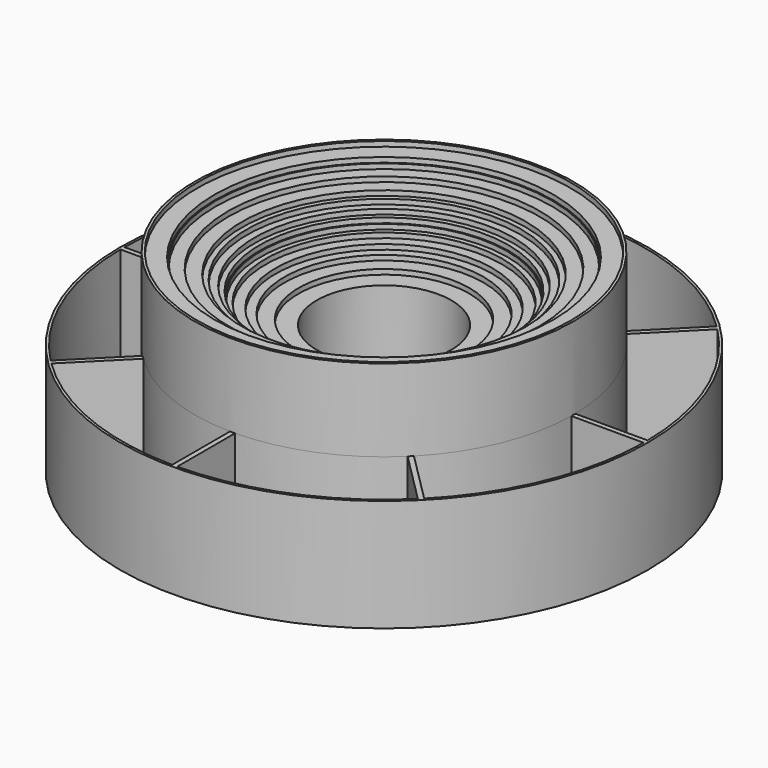
from build123d import *

# Parameters (mm, degrees)
F0_R      = 34.25
F0_R_2    = 27
F1_DEPTH  = 52
F2_R      = 40
F2_R_2    = 34.25
F3_DEPTH  = 54
F4_R      = 43.5
F4_R_2    = 40
F5_DEPTH  = 56
F6_R      = 47.5
F6_R_2    = 43.5
F7_DEPTH  = 58
F8_R      = 49.5
F8_R_2    = 47.5
F9_DEPTH  = 60
F10_R     = 50
F10_R_2   = 49.5
F11_DEPTH = 62
F12_R     = 52
F12_R_2   = 50
F13_DEPTH = 64
F14_R     = 55
F14_R_2   = 52
F15_DEPTH = 66
F16_R     = 57
F16_R_2   = 55
F17_DEPTH = 68
F18_R     = 62.5
F18_R_2   = 57
F19_DEPTH = 70
F20_R     = 67.5
F20_R_2   = 62.5
F21_DEPTH = 72
F22_R     = 68
F22_R_2   = 67.5
F23_DEPTH = 74
F24_R     = 75
F24_R_2   = 68
F25_DEPTH = 76
F26_R     = 76
F26_R_2   = 75
F27_DEPTH = 78
F29_DEPTH = 45
F30_R     = 106
F31_DEPTH = 45
F32_DEPTH = 40


# Not quite as in the source:
# - after a boolean that leaves OpenCascade's solid faulty, fix() repairs it


with BuildPart() as f1:
    # F0 (on Top) → F1 (new body)
    with BuildSketch(Plane.XY):
        Circle(F0_R)
        Circle(F0_R_2, mode=Mode.SUBTRACT)
    extrude(amount=F1_DEPTH)

    # F2 (on Top) → F3 (join)
    with BuildSketch(Plane.XY):
        Circle(F2_R)
        Circle(F2_R_2, mode=Mode.SUBTRACT)
    extrude(amount=F3_DEPTH)

    # F4 (on Top) → F5 (join)
    with BuildSketch(Plane.XY):
        Circle(F4_R)
        Circle(F4_R_2, mode=Mode.SUBTRACT)
    extrude(amount=F5_DEPTH)

    # F6 (on Top) → F7 (join)
    with BuildSketch(Plane.XY):
        Circle(F6_R)
        Circle(F6_R_2, mode=Mode.SUBTRACT)
    extrude(amount=F7_DEPTH)

    # F8 (on Top) → F9 (join)
    with BuildSketch(Plane.XY):
        Circle(F8_R)
        Circle(F8_R_2, mode=Mode.SUBTRACT)
    extrude(amount=F9_DEPTH)

    # F10 (on Top) → F11 (join)
    with BuildSketch(Plane.XY):
        Circle(F10_R)
        Circle(F10_R_2, mode=Mode.SUBTRACT)
    extrude(amount=F11_DEPTH)

    # F12 (on Top) → F13 (join)
    with BuildSketch(Plane.XY):
        Circle(F12_R)
        Circle(F12_R_2, mode=Mode.SUBTRACT)
    extrude(amount=F13_DEPTH)

    # F14 (on Top) → F15 (join)
    with BuildSketch(Plane.XY):
        Circle(F14_R)
        Circle(F14_R_2, mode=Mode.SUBTRACT)
    extrude(amount=F15_DEPTH)

    # F16 (on Top) → F17 (join)
    with BuildSketch(Plane.XY):
        Circle(F16_R)
        Circle(F16_R_2, mode=Mode.SUBTRACT)
    extrude(amount=F17_DEPTH)

    # F18 (on Top) → F19 (join)
    with BuildSketch(Plane.XY):
        Circle(F18_R)
        Circle(F18_R_2, mode=Mode.SUBTRACT)
    extrude(amount=F19_DEPTH)

    # F20 (on Top) → F21 (join)
    with BuildSketch(Plane.XY):
        Circle(F20_R)
        Circle(F20_R_2, mode=Mode.SUBTRACT)
    extrude(amount=F21_DEPTH)

    # F22 (on Top) → F23 (join)
    with BuildSketch(Plane.XY):
        Circle(F22_R)
        Circle(F22_R_2, mode=Mode.SUBTRACT)
    extrude(amount=F23_DEPTH)

    # F24 (on Top) → F25 (join)
    with BuildSketch(Plane.XY):
        Circle(F24_R)
        Circle(F24_R_2, mode=Mode.SUBTRACT)
    extrude(amount=F25_DEPTH)

    # F26 (on Top) → F27 (join)
    with BuildSketch(Plane.XY):
        Circle(F26_R)
        Circle(F26_R_2, mode=Mode.SUBTRACT)
    extrude(amount=F27_DEPTH)

    # F28 (on Top) → F29 (join)
    with BuildSketch(Plane.XY):
        with BuildLine():
            Line((105, 0), (76, 0))
            ThreePointArc((76, 0), (69.7127627842, -30.267651131), (51.8912972371, -55.5274100877))
            Line((51.8912972371, -55.5274100877), (72.4058930172, -76.0420058677))
            ThreePointArc((72.4058930172, -76.0420058677), (96.5080793685, -41.366539819), (105, 0))
        make_face()
        with BuildLine():
            ThreePointArc((55.5274100877, 51.8912972371), (70.6968286653, 27.8919059347), (76, 0))
            Line((76, 0), (105, 0))
            ThreePointArc((105, 0), (97.492078181, 38.9909565405), (76.0420058677, 72.4058930172))
            Line((76.0420058677, 72.4058930172), (55.5274100877, 51.8912972371))
        make_face()
        with BuildLine():
            ThreePointArc((0, 76), (30.267651131, 69.7127627842), (55.5274100877, 51.8912972371))
            Line((55.5274100877, 51.8912972371), (76.0420058677, 72.4058930172))
            ThreePointArc((76.0420058677, 72.4058930172), (41.366539819, 96.5080793685), (0, 105))
            Line((0, 105), (0, 76))
        make_face()
        with BuildLine():
            Line((72.4058930172, -76.0420058677), (51.8912972371, -55.5274100877))
            ThreePointArc((51.8912972371, -55.5274100877), (27.8919059347, -70.6968286653), (0, -76))
            Line((0, -76), (0, -105))
            ThreePointArc((0, -105), (38.9909565405, -97.492078181), (72.4058930172, -76.0420058677))
        make_face()
        with BuildLine():
            ThreePointArc((-51.8912972371, 55.5274100877), (-27.8919059347, 70.6968286653), (0, 76))
            Line((0, 76), (0, 105))
            ThreePointArc((0, 105), (-38.9909565405, 97.492078181), (-72.4058930172, 76.0420058677))
            Line((-72.4058930172, 76.0420058677), (-51.8912972371, 55.5274100877))
        make_face()
        with BuildLine():
            Line((0, -105), (0, -76))
            ThreePointArc((0, -76), (-30.267651131, -69.7127627842), (-55.5274100877, -51.8912972371))
            Line((-55.5274100877, -51.8912972371), (-76.0420058677, -72.4058930172))
            ThreePointArc((-76.0420058677, -72.4058930172), (-41.366539819, -96.5080793685), (0, -105))
        make_face()
        with BuildLine():
            ThreePointArc((-76, 0), (-69.7127627842, 30.267651131), (-51.8912972371, 55.5274100877))
            Line((-51.8912972371, 55.5274100877), (-72.4058930172, 76.0420058677))
            ThreePointArc((-72.4058930172, 76.0420058677), (-96.5080793685, 41.366539819), (-105, 0))
            Line((-105, 0), (-76, 0))
        make_face()
        with BuildLine():
            Line((-76.0420058677, -72.4058930172), (-55.5274100877, -51.8912972371))
            ThreePointArc((-55.5274100877, -51.8912972371), (-70.6968286653, -27.8919059347), (-76, 0))
            Line((-76, 0), (-105, 0))
            ThreePointArc((-105, 0), (-97.492078181, -38.9909565405), (-76.0420058677, -72.4058930172))
        make_face()
    extrude(amount=F29_DEPTH)

    # F30 (on face) → F31 (join)
    with BuildSketch(Plane.XY.offset(45)):
        Circle(F30_R)
        with BuildLine():
            ThreePointArc((74.9499515543, 73.5357379919), (97.0073509137, 40.1817603983), (104.9952379873, 1))
            ThreePointArc((104.9952379873, 1), (104.9988094901, 0.5000056692), (105, 0))
            ThreePointArc((105, 0), (104.9988094901, -0.5000056692), (104.9952379873, -1))
            ThreePointArc((104.9952379873, -1), (97.0073509137, -40.1817603983), (74.9499515543, -73.5357379919))
            ThreePointArc((74.9499515543, -73.5357379919), (74.2462120246, -74.2462120246), (73.5357379919, -74.9499515543))
            ThreePointArc((73.5357379919, -74.9499515543), (40.1817603983, -97.0073509137), (1, -104.9952379873))
            ThreePointArc((1, -104.9952379873), (0, -105), (-1, -104.9952379873))
            ThreePointArc((-1, -104.9952379873), (-40.1817603983, -97.0073509137), (-73.5357379919, -74.9499515543))
            ThreePointArc((-73.5357379919, -74.9499515543), (-74.2462120246, -74.2462120246), (-74.9499515543, -73.5357379919))
            ThreePointArc((-74.9499515543, -73.5357379919), (-97.0073509137, -40.1817603983), (-104.9952379873, -1))
            ThreePointArc((-104.9952379873, -1), (-105, 0), (-104.9952379873, 1))
            ThreePointArc((-104.9952379873, 1), (-97.0073509137, 40.1817603983), (-74.9499515543, 73.5357379919))
            ThreePointArc((-74.9499515543, 73.5357379919), (-74.2462120246, 74.2462120246), (-73.5357379919, 74.9499515543))
            ThreePointArc((-73.5357379919, 74.9499515543), (-40.1817603983, 97.0073509137), (-1, 104.9952379873))
            ThreePointArc((-1, 104.9952379873), (0, 105), (1, 104.9952379873))
            ThreePointArc((1, 104.9952379873), (40.1817603983, 97.0073509137), (73.5357379919, 74.9499515543))
            ThreePointArc((73.5357379919, 74.9499515543), (74.2462120246, 74.2462120246), (74.9499515543, 73.5357379919))
        make_face(mode=Mode.SUBTRACT)
    extrude(amount=-F31_DEPTH)

    # F30 (on face) → F32 (cut)
    with BuildSketch(Plane.XY.offset(45)):
        with BuildLine():
            Line((-74.9499515543, -73.5357379919), (-54.4425699317, -53.0283563693))
            ThreePointArc((-54.4425699317, -53.0283563693), (-70.2148444709, -29.0839408597), (-75.9934207679, -1))
            Line((-75.9934207679, -1), (-104.9952379873, -1))
            ThreePointArc((-104.9952379873, -1), (-97.0073509137, -40.1817603983), (-74.9499515543, -73.5357379919))
        make_face()
        with BuildLine():
            ThreePointArc((-75.9934207679, 1), (-70.2148444709, 29.0839408597), (-54.4425699317, 53.0283563693))
            Line((-54.4425699317, 53.0283563693), (-74.9499515543, 73.5357379919))
            ThreePointArc((-74.9499515543, 73.5357379919), (-97.0073509137, 40.1817603983), (-104.9952379873, 1))
            Line((-104.9952379873, 1), (-75.9934207679, 1))
        make_face()
        with BuildLine():
            ThreePointArc((-53.0283563693, 54.4425699317), (-29.0839408597, 70.2148444709), (-1, 75.9934207679))
            Line((-1, 75.9934207679), (-1, 104.9952379873))
            ThreePointArc((-1, 104.9952379873), (-40.1817603983, 97.0073509137), (-73.5357379919, 74.9499515543))
            Line((-73.5357379919, 74.9499515543), (-53.0283563693, 54.4425699317))
        make_face()
        with BuildLine():
            ThreePointArc((1, 75.9934207679), (29.0839408597, 70.2148444709), (53.0283563693, 54.4425699317))
            Line((53.0283563693, 54.4425699317), (73.5357379919, 74.9499515543))
            ThreePointArc((73.5357379919, 74.9499515543), (40.1817603983, 97.0073509137), (1, 104.9952379873))
            Line((1, 104.9952379873), (1, 75.9934207679))
        make_face()
        with BuildLine():
            ThreePointArc((54.4425699317, 53.0283563693), (70.2148444709, 29.0839408597), (75.9934207679, 1))
            Line((75.9934207679, 1), (104.9952379873, 1))
            ThreePointArc((104.9952379873, 1), (97.0073509137, 40.1817603983), (74.9499515543, 73.5357379919))
            Line((74.9499515543, 73.5357379919), (54.4425699317, 53.0283563693))
        make_face()
        with BuildLine():
            Line((104.9952379873, -1), (75.9934207679, -1))
            ThreePointArc((75.9934207679, -1), (70.2148444709, -29.0839408597), (54.4425699317, -53.0283563693))
            Line((54.4425699317, -53.0283563693), (74.9499515543, -73.5357379919))
            ThreePointArc((74.9499515543, -73.5357379919), (97.0073509137, -40.1817603983), (104.9952379873, -1))
        make_face()
        with BuildLine():
            Line((73.5357379919, -74.9499515543), (53.0283563693, -54.4425699317))
            ThreePointArc((53.0283563693, -54.4425699317), (29.0839408597, -70.2148444709), (1, -75.9934207679))
            Line((1, -75.9934207679), (1, -104.9952379873))
            ThreePointArc((1, -104.9952379873), (40.1817603983, -97.0073509137), (73.5357379919, -74.9499515543))
        make_face()
        with BuildLine():
            Line((-1, -104.9952379873), (-1, -75.9934207679))
            ThreePointArc((-1, -75.9934207679), (-29.0839408597, -70.2148444709), (-53.0283563693, -54.4425699317))
            Line((-53.0283563693, -54.4425699317), (-73.5357379919, -74.9499515543))
            ThreePointArc((-73.5357379919, -74.9499515543), (-40.1817603983, -97.0073509137), (-1, -104.9952379873))
        make_face()
    extrude(amount=-F32_DEPTH, mode=Mode.SUBTRACT)

    add(f1.part.fix(), mode=Mode.REPLACE)


solid = f1.part
